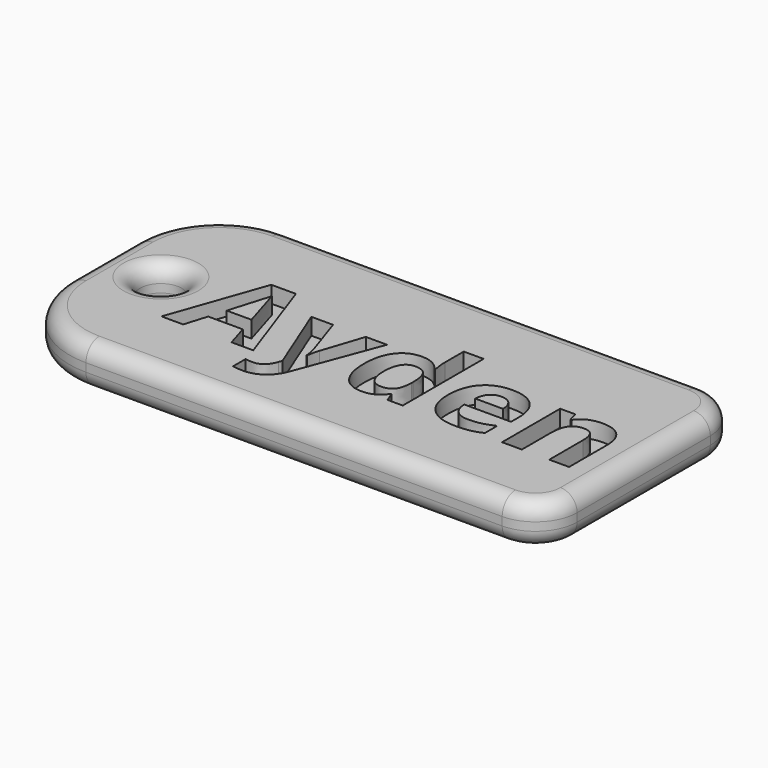
from build123d import *

# Parameters (mm, degrees)
F0_W         = 65
F0_H         = 30
F1_DEPTH     = 5
F2_R         = 2.5
F3_DEPTH     = 5.001
F4_R         = 5
F5_R         = 10
F6_TEXT_SIZE = 15.9776313162
F7_DEPTH     = 2
F8_R         = 2


# Not quite as in the source:
# - Text() gives the source's letters only with a copy of the font that has no kerning and outlines rounded to 1/6400 em; it was checked with that copy


with BuildPart() as f1:
    # F0 (on Top) → F1 (new body)
    with BuildSketch(Plane.XY):
        with Locations((32.5, 15)):
            Rectangle(F0_W, F0_H)
    extrude(amount=F1_DEPTH)

    # F2 (on face) → F3 (cut, through all)
    with BuildSketch(Plane.XY.offset(5)):
        with Locations((7, 15)):
            Circle(F2_R)
    extrude(amount=-F3_DEPTH, mode=Mode.SUBTRACT)

    # F4
    f4_edges = [f1.edges().sort_by_distance(p)[0] for p in [
        (65, 30, 2.5),
        (65, 0, 2.5),
    ]]
    fillet(f4_edges, radius=F4_R)

    # F5
    f5_edges = [f1.edges().sort_by_distance(p)[0] for p in [
        (0, 30, 2.5),
        (0, 0, 2.5),
    ]]
    fillet(f5_edges, radius=F5_R)

    # F6 (on face) → F7 (cut)
    with BuildSketch(Plane.XY.offset(5)):
        with Locations((12.0522799005, 8.7738210157)):
            Text('Ayden', F6_TEXT_SIZE, font='Open Sans', font_style=FontStyle.BOLD, text_align=(TextAlign.LEFT, TextAlign.BOTTOM))
    extrude(amount=-F7_DEPTH, mode=Mode.SUBTRACT)

    # F8
    f8_edges = [f1.edges().sort_by_distance(p)[0] for p in [
        (35, 30, 5),
        (63.535534, 28.535534, 5),
        (35, 30, 0),
        (2.928932, 27.071068, 0),
        (63.535534, 28.535534, 0),
        (0, 15, 0),
        (65, 15, 0),
        (2.928932, 2.928932, 0),
        (63.535534, 1.464466, 0),
        (35, 0, 0),
        (4.5, 15, 0),
        (4.5, 15, 5),
    ]]
    fillet(f8_edges, radius=F8_R)


solid = f1.part
